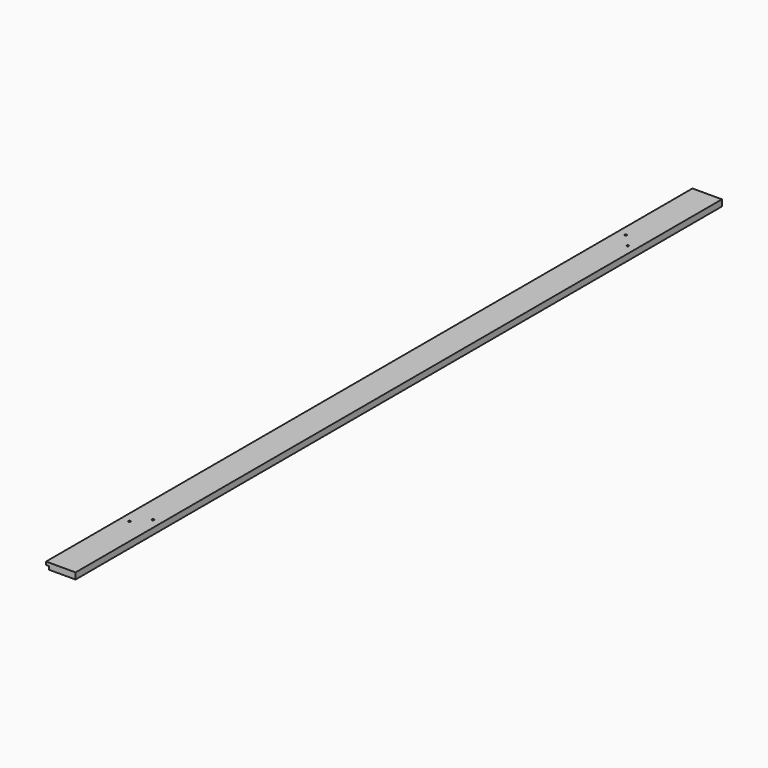
from build123d import *

# Parameters (mm, degrees)
F0_W     = 88.9
F0_H     = 19.05
F1_DEPTH = 1219.2
F2_W     = 16.1721451446
F2_H     = 19.628858405
F3_DEPTH = 3660
F4_R     = 3.175
F5_DEPTH = 19.05


# Not quite as in the source:
# - an extrude ends at something that could not be found from the text; its depth is read off the source's solid


with BuildPart() as f1:
    # F0 (on Front) → F1 (new body, symmetric)
    with BuildSketch(Plane.XZ):
        Rectangle(F0_W, F0_H)
    extrude(amount=F1_DEPTH, both=True)

    # F2 (on face) → F3 (cut, through all)
    with BuildSketch(Plane.XZ.offset(1219.2)):
        with Locations((-43.0110725723, -9.8144292025)):
            Rectangle(F2_W, F2_H)
    extrude(amount=-F3_DEPTH, mode=Mode.SUBTRACT)

    # F4 (on face) → F5 (cut, through all)
    with BuildSketch(Plane.XY.offset(9.525)):
        with Locations((19.05, -895.35)):
            Circle(F4_R)
        with Locations((-19.05, -935.99)):
            Circle(F4_R)
        with Locations((-19.05, 935.99)):
            Circle(F4_R)
        with Locations((19.05, 895.35)):
            Circle(F4_R)
    extrude(amount=-F5_DEPTH, mode=Mode.SUBTRACT)


solid = f1.part
